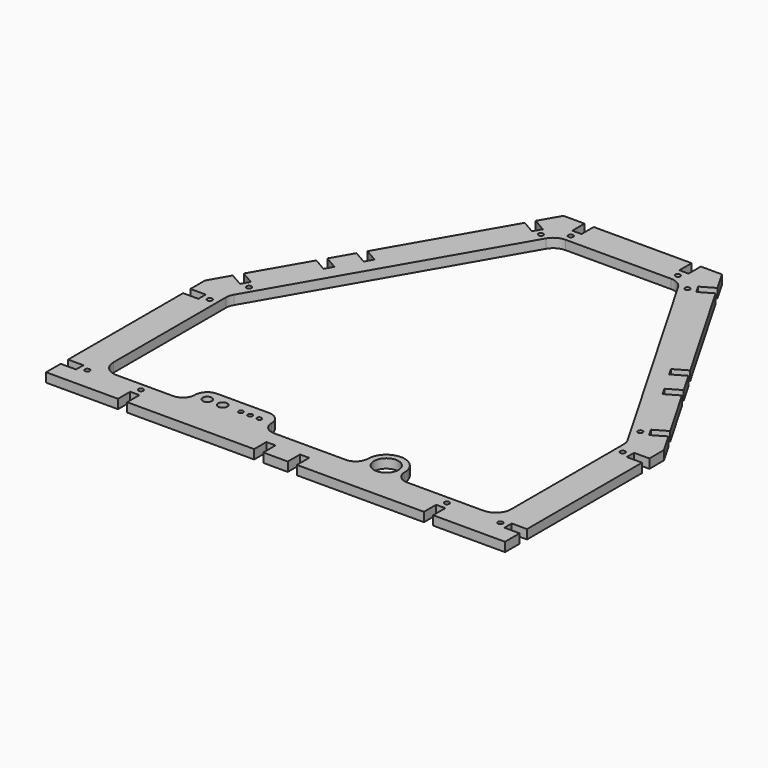
from build123d import *

# Parameters (mm, degrees)
F1_DEPTH  = 6
F2_R      = 1.6
F2_W      = 10
F2_H      = 6
F2_W_2    = 6
F2_H_2    = 10
F3_DEPTH  = 6.001
F4_W      = 6
F4_H      = 10
F5_DEPTH  = 6.001
F7_DEPTH  = 6.001
F8_R      = 10
F9_R      = 8
F9_R_2    = 3
F9_R_3    = 1.5
F10_DEPTH = 6.001
F11_R     = 7.99999


# Not quite as in the source:
# - a fillet or chamfer is up to 0.001 mm smaller than in the source, because OpenCascade refuses the exact size


with BuildPart() as f1:
    # F0 (on Top) → F1 (new body)
    with BuildSketch(Plane.XY):
        Polygon((-150, -150), (150, -150), (150, -20.0961894323), (51.7949192431, 150), (-51.7949192431, 150), (-150, -20.0961894323), align=None)
    extrude(amount=F1_DEPTH)

    # F2 (on face) → F3 (cut, through all)
    with BuildSketch(Plane.XY.offset(6)):
        Polygon((-139.3974596216, -1.7320508076), (-142.3974596216, -6.9282032303), (-133.7372055837, -11.9282032303), (-130.7372055837, -6.7320508076), align=None)
        with Locations((-127.9070785648, -11.8301270189)):
            Circle(F2_R)
        Polygon((-50.7372055837, 131.8320137979), (-59.3974596216, 136.8320137979), (-62.3974596216, 131.6358613752), (-53.7372055837, 126.6358613752), align=None)
        with Locations((-47.9070785648, 126.7339375866)):
            Circle(F2_R)
        Polygon((133.7372055837, -11.9282032303), (142.3974596216, -6.9282032303), (139.3974596216, -1.7320508076), (130.7372055837, -6.7320508076), align=None)
        with Locations((127.9070785648, -11.8301270189)):
            Circle(F2_R)
        Polygon((53.7372055837, 126.6358613752), (62.3974596216, 131.6358613752), (59.3974596216, 136.8320137979), (50.7372055837, 131.8320137979), align=None)
        with Locations((47.9070785648, 126.7339375866)):
            Circle(F2_R)
        with Locations((-145, -35.0480947162)):
            Rectangle(F2_W, F2_H)
        with Locations((-135, -35.0480947162)):
            Circle(F2_R)
        with Locations((-145, -135.0480947162)):
            Rectangle(F2_W, F2_H)
        with Locations((-135, -135.0480947162)):
            Circle(F2_R)
        with Locations((145, -135.0480947162)):
            Rectangle(F2_W, F2_H)
        with Locations((135, -135.0480947162)):
            Circle(F2_R)
        with Locations((135, -35.0480947162)):
            Circle(F2_R)
        with Locations((145, -35.0480947162)):
            Rectangle(F2_W, F2_H)
        with Locations((-35, 145)):
            Rectangle(F2_W_2, F2_H_2)
        with Locations((-35, 135)):
            Circle(F2_R)
        with Locations((35, 145)):
            Rectangle(F2_W_2, F2_H_2)
        with Locations((35, 135)):
            Circle(F2_R)
        with Locations((-100, -145)):
            Rectangle(F2_W_2, F2_H_2)
        with Locations((-100, -135)):
            Circle(F2_R)
        with Locations((100, -135)):
            Circle(F2_R)
        with Locations((100, -145)):
            Rectangle(F2_W_2, F2_H_2)
    extrude(amount=-F3_DEPTH, mode=Mode.SUBTRACT)

    # F4 (on face) → F5 (cut, through all)
    with BuildSketch(Plane.XY.offset(6)):
        with Locations((-11, -145)):
            Rectangle(F4_W, F4_H)
        with Locations((11, -145)):
            Rectangle(F4_W, F4_H)
        Polygon((-107.8397459622, 32.9275126212), (-116.5, 37.9275126212), (-119.5, 32.7313601985), (-110.8397459622, 27.7313601985), align=None)
        Polygon((-105.5, 56.9800715045), (-108.5, 51.7839190818), (-99.8397459622, 46.7839190818), (-96.8397459622, 51.9800715045), align=None)
        Polygon((107.8397459622, 32.9275126212), (110.8397459622, 27.7313601985), (119.5, 32.7313601985), (116.5, 37.9275126212), align=None)
        Polygon((105.5, 56.9800715045), (96.8397459622, 51.9800715045), (99.8397459622, 46.7839190818), (108.5, 51.7839190818), align=None)
    extrude(amount=-F5_DEPTH, mode=Mode.SUBTRACT)

    # F6 (on face) → F7 (cut, through all)
    with BuildSketch(Plane.XY.offset(6)):
        with BuildLine():
            Line((62, -130), (130, -130))
            Line((130, -130), (130, -25.455173281))
            Line((130, -25.455173281), (40.2479138593, 130))
            Line((40.2479138593, 130), (-40.2479138593, 130))
            Line((-40.2479138593, 130), (-130, -25.455173281))
            Line((-130, -25.455173281), (-130, -130))
            Line((-130, -130), (-75, -130))
            Line((-75, -130), (-75, -114))
            Line((-75, -114), (-25, -114))
            Line((-25, -114), (-25, -130))
            Line((-25, -130), (38, -130))
            Line((38, -130), (38, -122))
            ThreePointArc((38, -122), (50, -110), (62, -122))
            Line((62, -122), (62, -130))
        make_face()
    extrude(amount=-F7_DEPTH, mode=Mode.SUBTRACT)

    # F8
    f8_edges = [f1.edges().sort_by_distance(p)[0] for p in [
        (-40.247914, 130, 3),
        (-130, -25.455173, 3),
        (130, -25.455173, 3),
        (40.247914, 130, 3),
        (130, -130, 3),
        (-130, -130, 3),
    ]]
    fillet(f8_edges, radius=F8_R)

    # F9 (on face) → F10 (cut, through all)
    with BuildSketch(Plane.XY.offset(6)):
        with Locations((50, -122)):
            Circle(F9_R)
        with Locations((-67, -122)):
            Circle(F9_R_2)
        with Locations((-57, -122)):
            Circle(F9_R_2)
        with Locations((-39, -122)):
            Circle(F9_R_3)
        with Locations((-33, -122)):
            Circle(F9_R_3)
        with Locations((-45, -122)):
            Circle(F9_R_3)
    extrude(amount=-F10_DEPTH, mode=Mode.SUBTRACT)

    # F11 (radius 8 in the source; OpenCascade refuses exactly that, so slightly less here)
    f11_edges = [f1.edges().sort_by_distance(p)[0] for p in [
        (-75, -130, 3),
        (-75, -114, 3),
        (-25, -114, 3),
        (-25, -130, 3),
        (62, -130, 3),
        (38, -130, 3),
    ]]
    fillet(f11_edges, radius=F11_R)


solid = f1.part
